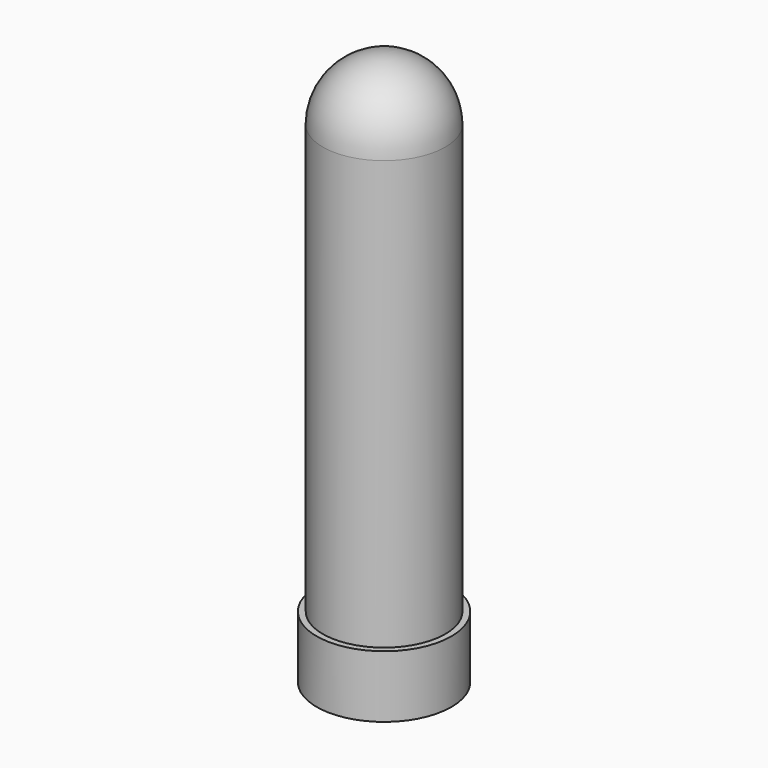
from build123d import *

# Parameters (mm, degrees)
F2_R     = 27.5
F2_R_2   = 25
F3_DEPTH = 25.4
F4_DEPTH = 8
F5_R     = 2
F6_DEPTH = 25


with BuildPart() as f1:
    # F0 (on Right) → F1 (revolve)
    with BuildSketch(Plane.YZ):
        with BuildLine():
            Line((0, 200), (0, 0))
            Line((0, 0), (25, 0))
            Line((25, 0), (25, 175))
            ThreePointArc((25, 175), (17.6776695297, 192.6776695297), (0, 200))
        make_face()
    revolve(axis=Axis((0, 0, 100), (0, 0, 1)))


with BuildPart() as f3:
    # F2 (on Top) → F3 (new body)
    with BuildSketch(Plane.XY):
        Circle(F2_R)
        Circle(F2_R_2, mode=Mode.SUBTRACT)
    extrude(amount=-F3_DEPTH)

    # F2 (on Top) → F4 (join)
    with BuildSketch(Plane.XY):
        Circle(F2_R_2)
    extrude(amount=-F4_DEPTH)

    # F5 (on face) → F6 (cut)
    with BuildSketch(Plane.XY):
        with BuildLine():
            ThreePointArc((9.9148839653, 6.0952902816), (7.2703518936, 7.98858857), (6.3303055567, 4.8749988135))
            ThreePointArc((6.3303055567, 4.8749988135), (8.559416037, 4.2019919933), (9.9148839653, 6.0952902816))
        make_face()
        with BuildLine():
            ThreePointArc((-17.8055719167, 2.7819635249), (-21.8007052936, 2.921400996), (-17.825014725, 2.5037671724))
            ThreePointArc((-17.825014725, 2.5037671724), (-17.8104385397, 2.6425260539), (-17.8055719167, 2.7819635249))
        make_face()
        with BuildLine():
            ThreePointArc((-7.9859973724, -0.2789413551), (-8.1615739108, 0.5404968871), (-8.6574764052, 1.2160609993))
            Line((-8.6574764052, 1.2160609993), (-10.851248059, 1.5242062399))
            ThreePointArc((-10.851248059, 1.5242062399), (-11.0512435005, -1.9716464938), (-7.9859973724, -0.2789413551))
        make_face()
        with BuildLine():
            Line((-10.851248059, 1.5242062399), (-8.6574764052, 1.2160609993))
            ThreePointArc((-8.6574764052, 1.2160609993), (-9.7078010199, 1.7016158366), (-10.851248059, 1.5242062399))
        make_face()
        with Locations((-15.971799481, -12.0375089341)):
            Circle(F5_R)
        with Locations((-2.7819635249, -19.8055719167)):
            Circle(F5_R)
        with Locations((12.0375089341, -15.971799481)):
            Circle(F5_R)
        with Locations((19.8055719167, -2.7819635249)):
            Circle(F5_R)
        with Locations((15.971799481, 12.0375089341)):
            Circle(F5_R)
        with Locations((2.7819635249, 19.8055719167)):
            Circle(F5_R)
        with Locations((-12.0375089341, 15.971799481)):
            Circle(F5_R)
        with Locations((-3.3511318873, 9.4110502536)):
            Circle(F5_R)
        with Locations((-2.8205539004, -9.5834454919)):
            Circle(F5_R)
        with Locations((8.2427991948, -5.6439536882)):
            Circle(F5_R)
    extrude(amount=-F6_DEPTH, mode=Mode.SUBTRACT)


solid = Compound([f1.part, f3.part])
